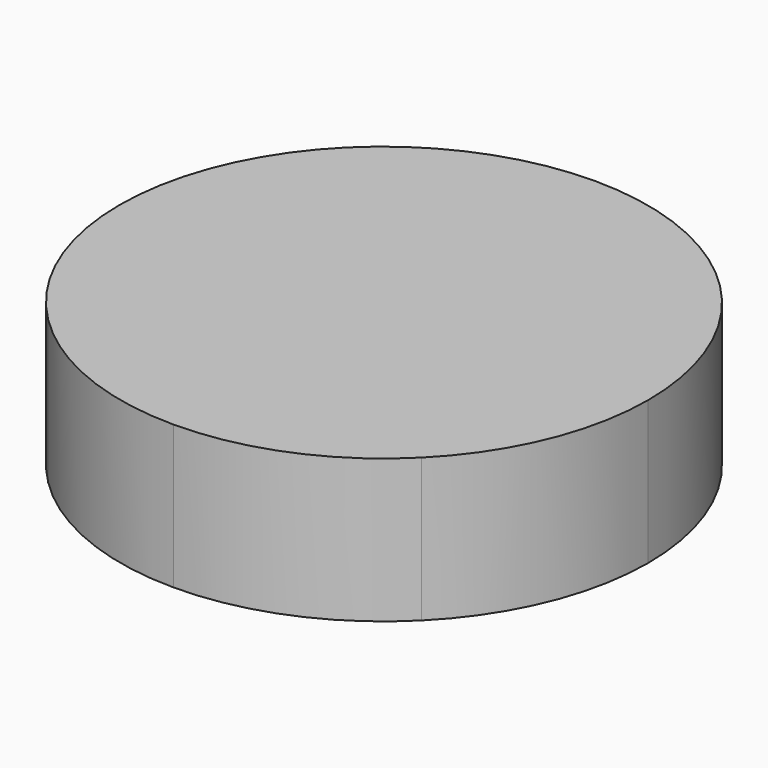
from build123d import *

# Parameters (mm, degrees)
F3_W     = 421.7902910393
F3_H     = 198.2180179606
F4_DEPTH = 25.4


# Not quite as in the source:
# - ends of sketch curves that miss each other by under 0.0002 mm in the source are joined


with BuildPart() as f1:
    # F0 (on Front) → F1 (revolve)
    with BuildSketch(Plane.XZ):
        with BuildLine():
            Line((10.5788812285, 8.2366884696), (-24.2557799278, 8.2366884696))
            Line((-24.2557799278, 8.2366884696), (-24.6392214836, 8.2366884696))
            ThreePointArc((-24.6392214836, 8.2366884696), (-32.6864160689, -0.0082121834), (-24.6228011914, -8.2370543))
            Line((-24.6228011914, -8.2370543), (-24.27220022, -8.2370543))
            Line((-24.27220022, -8.2370543), (10.5788812285, -8.2370543))
            Line((10.5788812285, -8.2370543), (10.5788812285, 8.2366884696))
        make_face()
    revolve(axis=Axis((10.5788812285, 0, -0.0001829152), (0, 0, -1)))

    # F3 (on offset) → F4 (cut)
    with BuildSketch(Plane.XY.offset(10)):
        Rectangle(F3_W, F3_H)
        with BuildLine():
            ThreePointArc((-10.7153009133, 20.1523680538), (-0.8347905086, 26.6913979084), (10.7887436299, 28.9885377447))
            ThreePointArc((10.7887436299, 28.9885377447), (22.3773621495, 26.6792950108), (32.203329708, 20.1158334422))
            ThreePointArc((32.203329708, 20.1158334422), (38.769051111, 10.2908037813), (41.0760354322, -1.2987526262))
            ThreePointArc((41.0760354322, -1.2987526262), (38.7450627408, -12.8738402066), (32.1768729102, -22.6858234277))
            ThreePointArc((32.1768729102, -22.6858234277), (22.3718072579, -29.2722876696), (10.7887436292, -31.5860449158))
            ThreePointArc((10.7887436292, -31.5860449158), (-0.8256146846, -29.2802975648), (-10.6861755573, -22.7244524913))
            ThreePointArc((-10.6861755573, -22.7244524913), (-17.3142524075, -12.9103633574), (-19.6419716109, -1.2987526263))
            ThreePointArc((-19.6419716109, -1.2987526263), (-17.3228833961, 10.3191134223), (-10.7153009133, 20.1523680538))
        make_face(mode=Mode.SUBTRACT)
    extrude(amount=-F4_DEPTH, mode=Mode.SUBTRACT)


solid = f1.part
